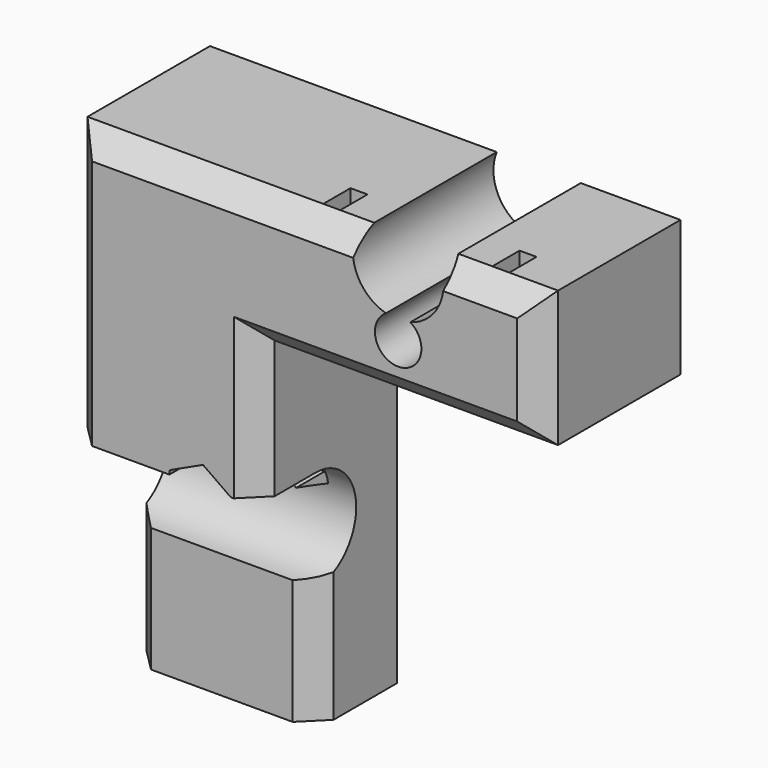
from build123d import *

# Parameters (mm, degrees)
F1_DEPTH  = 17.5
F2_W      = 16.5
F2_H      = 20
F3_DEPTH  = 11
F4_R      = 1.75
F6_DEPTH  = 22.5
F8_DEPTH  = 7.5
F9_DEPTH  = 13.1
F10_DEPTH = 24.9
F11_R     = 1.75
F12_DEPTH = 2
F13_W     = 15.5
F13_H     = 6.6
F13_H_2   = 5.4
F14_DEPTH = 25
F15_DEPTH = 16.5
F17_DEPTH = 25
F18_W     = 1.5
F18_H     = 3
F19_DEPTH = 25
F21_DEPTH = 15.5
F22_SIZE  = 1.99999
F23_SIZE  = 2


# Not quite as in the source:
# - a fillet or chamfer is up to 0.001 mm smaller than in the source, because OpenCascade refuses the exact size


with BuildPart() as f1:
    # F0 (on Front) → F1 (new body)
    with BuildSketch(Plane.XZ):
        with BuildLine():
            Line((16.5, 21), (16.5, 21.3678174192))
            Line((16.5, 21.3678174192), (16.5, 38.5))
            Line((16.5, 38.5), (11.9580992435, 38.5))
            ThreePointArc((11.9580992435, 38.5), (11.8488094961, 35.2539844758), (9.3668783978, 33.1590909091))
            ThreePointArc((9.3668783978, 33.1590909091), (8.25, 29.3900555271), (7.1331216022, 33.1590909091))
            ThreePointArc((7.1331216022, 33.1590909091), (4.6511905039, 35.2539844758), (4.5419007565, 38.5))
            Line((4.5419007565, 38.5), (0, 38.5))
            Line((0, 38.5), (0, 21.3678174192))
            Line((0, 21.3678174192), (0, 21))
            Line((0, 21), (8.25, 21))
            Line((8.25, 21), (16.5, 21))
        make_face()
    extrude(amount=F1_DEPTH)

    # F2 (on face) → F3 (join)
    with BuildSketch(Plane(origin=(0, 0, 0), x_dir=(-1, 0, 0), z_dir=(0, 1, 0))):
        with Locations((-8.25, 11)):
            Rectangle(F2_W, F2_H)
    extrude(amount=-F3_DEPTH)

    # F4 (on face) → F6 (cut)
    with BuildSketch(Plane(origin=(0, 0, 0), x_dir=(-1, 0, 0), z_dir=(0, 1, 0))):
        with Locations((-11.5, 19.5)):
            Circle(F4_R)
    extrude(amount=-F6_DEPTH, mode=Mode.SUBTRACT)

    # F7 (on face) → F8 (cut)
    with BuildSketch(Plane.XZ.offset(11)):
        Polygon((14.1428062528, 17.6374994111), (14.4343759509, 20.8574870578), (11.7915696981, 22.7199876466), (8.8571937472, 21.3625005889), (8.5656240491, 18.1425129422), (11.2084303019, 16.2800123534), align=None)
    extrude(amount=-F8_DEPTH, mode=Mode.SUBTRACT)

    # F7 (on face) → F9 (cut)
    with BuildSketch(Plane.XZ.offset(11)):
        Polygon((14.1428062528, 17.6374994111), (14.4343759509, 20.8574870578), (11.7915696981, 22.7199876466), (8.8571937472, 21.3625005889), (8.5656240491, 18.1425129422), (11.2084303019, 16.2800123534), align=None)
    extrude(amount=F9_DEPTH, mode=Mode.SUBTRACT)

    # F5 (on face) → F10 (cut)
    with BuildSketch(Plane(origin=(0, 0, 0), x_dir=(0, -1, 0), z_dir=(-1, 0, 0))):
        with BuildLine():
            Line((11, 16.5), (11, 21))
            ThreePointArc((11, 21), (6.5, 16.5), (11, 12))
            Line((11, 12), (11, 16.5))
        make_face()
    extrude(amount=-F10_DEPTH, mode=Mode.SUBTRACT)

    # F11 (on face) → F12 (cut)
    with BuildSketch(Plane(origin=(0, 0, 0), x_dir=(-1, 0, 0), z_dir=(0, 1, 0))):
        with BuildLine():
            Line((-11.9580992435, 38.5), (-16.5, 38.5))
            Line((-16.5, 38.5), (-16.5, 1))
            Line((-16.5, 1), (0, 1))
            Line((0, 1), (0, 38.5))
            Line((0, 38.5), (-4.5419007565, 38.5))
            ThreePointArc((-4.5419007565, 38.5), (-4.6511905039, 35.2539844758), (-7.1331216022, 33.1590909091))
            ThreePointArc((-7.1331216022, 33.1590909091), (-8.25, 29.3900555271), (-9.3668783978, 33.1590909091))
            ThreePointArc((-9.3668783978, 33.1590909091), (-11.8488094961, 35.2539844758), (-11.9580992435, 38.5))
        make_face()
        with Locations((-11.5, 19.5)):
            Circle(F11_R, mode=Mode.SUBTRACT)
    extrude(amount=-F12_DEPTH, mode=Mode.SUBTRACT)

    # F13 (on face) → F14 (join)
    with BuildSketch(Plane.YZ.offset(16.5)):
        with Locations((-9.75, 41.8)):
            Rectangle(F13_W, F13_H)
        with Locations((-9.75, 35.8)):
            Rectangle(F13_W, F13_H_2)
    extrude(amount=F14_DEPTH)

    # F15 (add): a face of the model
    f15_faces = [f1.faces().sort_by_distance(p)[0] for p in [
        (16.5, -9.75, 41.8),
    ]]
    extrude(f15_faces, amount=F15_DEPTH)

    # F16 (on face) → F17 (cut)
    with BuildSketch(Plane(origin=(0, -2, 0), x_dir=(-1, 0, 0), z_dir=(0, 1, 0))):
        with BuildLine():
            ThreePointArc((-30.0731763785, 39.739389973), (-29, 35.9427381873), (-27.9268236215, 39.739389973))
            ThreePointArc((-27.9268236215, 39.739389973), (-25.4094368312, 41.8298269216), (-25.2948465851, 45.1))
            Line((-25.2948465851, 45.1), (-32.7051534149, 45.1))
            ThreePointArc((-32.7051534149, 45.1), (-32.5905631688, 41.8298269216), (-30.0731763785, 39.739389973))
        make_face()
    extrude(amount=-F17_DEPTH, mode=Mode.SUBTRACT)

    # F18 (on face) → F19 (cut)
    with BuildSketch(Plane.XY.offset(45.1)):
        with Locations((21.5448465851, -14)):
            Rectangle(F18_W, F18_H)
        with Locations((36.4551534149, -14)):
            Rectangle(F18_W, F18_H)
    extrude(amount=-F19_DEPTH, mode=Mode.SUBTRACT)

    # F20 (on face) → F21 (join)
    with BuildSketch(Plane.XZ.offset(17.5)):
        with BuildLine():
            Line((10.089985095, 38.5), (10.0875691268, 38.5))
            Line((10.0875691268, 38.5), (4.5419007565, 38.5))
            ThreePointArc((4.5419007565, 38.5), (4.6511905039, 35.2539844758), (7.1331216022, 33.1590909091))
            ThreePointArc((7.1331216022, 33.1590909091), (8.25, 29.3900555271), (9.3668783978, 33.1590909091))
            ThreePointArc((9.3668783978, 33.1590909091), (11.8488094961, 35.2539844758), (11.9580992435, 38.5))
            Line((11.9580992435, 38.5), (10.089985095, 38.5))
        make_face()
    extrude(amount=-F21_DEPTH)

    # F22 (size 2 in the source; OpenCascade refuses exactly that, so slightly less here)
    f22_edges = [f1.edges().sort_by_distance(p)[0] for p in [
        (41.5, -17.5, 39.1),
        (0, -17.5, 33.05),
        (16.5, -17.5, 27.05),
        (29, -17.5, 33.1),
        (12.647423, -17.5, 45.1),
        (37.102577, -17.5, 45.1),
    ]]
    chamfer(f22_edges, length=F22_SIZE)

    # F23
    f23_edges = [f1.edges().sort_by_distance(p)[0] for p in [
        (0, -11, 6.5),
        (16.5, -11, 6.5),
    ]]
    chamfer(f23_edges, length=F23_SIZE)


solid = f1.part
